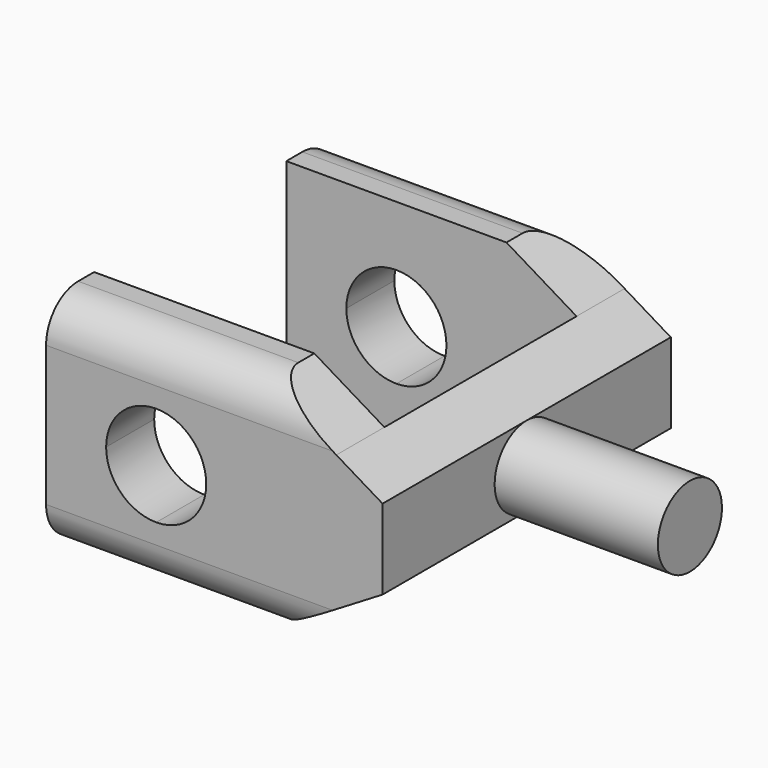
from build123d import *

# Parameters (mm, degrees)
F3_W     = 8.1543137785
F3_H     = 2
F5_DEPTH = 9
F6_DEPTH = 6
F8_R     = 2


# Not quite as in the source:
# - a feature names something its author has since deleted; it is built from what else it names


with BuildPart() as f4:
    # F3 (on Front) → F4 (revolve)
    with BuildSketch(Plane.XZ):
        with Locations((6.3856310444, -2.5)):
            Rectangle(F3_W, F3_H)
    revolve(axis=Axis((6.3856310444, 0, -1.5), (1, 0, 0)))

    # F3 (on Front) → F5 (join, symmetric)
    with BuildSketch(Plane.XZ):
        with BuildLine():
            ThreePointArc((-9, 1), (-7.232233047, 0.267766953), (-6.5, -1.5))
            Line((-6.5, -1.5), (-3.5, -1.5))
            Line((-3.5, -1.5), (-3.5, 4))
            Line((-3.5, 4), (-9, 4))
            Line((-9, 4), (-9, 1))
        make_face()
        with BuildLine():
            Line((-3.5, -1.5), (-6.5, -1.5))
            ThreePointArc((-6.5, -1.5), (-7.232233047, -3.267766953), (-9, -4))
            Line((-9, -4), (-9, -7))
            Line((-9, -7), (-3.5, -7))
            Line((-3.5, -7), (-3.5, -1.5))
        make_face()
        with BuildLine():
            Line((-9, -7), (-9, -4))
            ThreePointArc((-9, -4), (-10.767766953, -3.267766953), (-11.5, -1.5))
            Line((-11.5, -1.5), (-14.5, -1.5))
            Line((-14.5, -1.5), (-14.5, -7))
            Line((-14.5, -7), (-9, -7))
        make_face()
        with BuildLine():
            ThreePointArc((-11.5, -1.5), (-10.767766953, 0.267766953), (-9, 1))
            Line((-9, 1), (-9, 4))
            Line((-9, 4), (-14.5, 4))
            Line((-14.5, 4), (-14.5, -1.5))
            Line((-14.5, -1.5), (-11.5, -1.5))
        make_face()
        Polygon((0, 1.8910123945), (0, -1.5), (2.3084741551, -1.5), (2.3084741551, 0.5), align=None)
        Polygon((2.3084741551, -1.5), (0, -1.5), (0, -4.8910123945), (2.3084741551, -3.5), align=None)
        Polygon((-3.5, 4), (-3.5, -1.5), (0, -1.5), (0, 1.8910123945), align=None)
        Polygon((0, -1.5), (-3.5, -1.5), (-3.5, -7), (0, -4.8910123945), align=None)
    extrude(amount=F5_DEPTH, both=True)


with BuildPart() as f6:
    # F3 (on Front) → F6 (new body, symmetric)
    with BuildSketch(Plane.XZ):
        with BuildLine():
            ThreePointArc((-11.5, -1.5), (-10.767766953, 0.267766953), (-9, 1))
            Line((-9, 1), (-9, 4))
            Line((-9, 4), (-14.5, 4))
            Line((-14.5, 4), (-14.5, -1.5))
            Line((-14.5, -1.5), (-11.5, -1.5))
        make_face()
        with BuildLine():
            ThreePointArc((-9, 1), (-7.232233047, 0.267766953), (-6.5, -1.5))
            Line((-6.5, -1.5), (-3.5, -1.5))
            Line((-3.5, -1.5), (-3.5, 4))
            Line((-3.5, 4), (-9, 4))
            Line((-9, 4), (-9, 1))
        make_face()
        with BuildLine():
            Line((-3.5, -1.5), (-6.5, -1.5))
            ThreePointArc((-6.5, -1.5), (-7.232233047, -3.267766953), (-9, -4))
            Line((-9, -4), (-9, -7))
            Line((-9, -7), (-3.5, -7))
            Line((-3.5, -7), (-3.5, -1.5))
        make_face()
        with BuildLine():
            Line((-9, -7), (-9, -4))
            ThreePointArc((-9, -4), (-10.767766953, -3.267766953), (-11.5, -1.5))
            Line((-11.5, -1.5), (-14.5, -1.5))
            Line((-14.5, -1.5), (-14.5, -7))
            Line((-14.5, -7), (-9, -7))
        make_face()
        Polygon((-3.5, 4), (-3.5, -1.5), (0, -1.5), (0, 1.8910123945), align=None)
        Polygon((0, -1.5), (-3.5, -1.5), (-3.5, -7), (0, -4.8910123945), align=None)
    extrude(amount=F6_DEPTH, both=True)


with BuildPart() as f4_1:
    add(f4.part)

    # F7: cut F6
    add(f6.part, mode=Mode.SUBTRACT)

    # F8
    f8_edges = [f4_1.edges().sort_by_distance(p)[0] for p in [
        (-9, -9, 4),
        (-9, -9, -7),
        (-9, 9, -7),
        (-9, 9, 4),
    ]]
    fillet(f8_edges, radius=F8_R)


solid = f4_1.part
